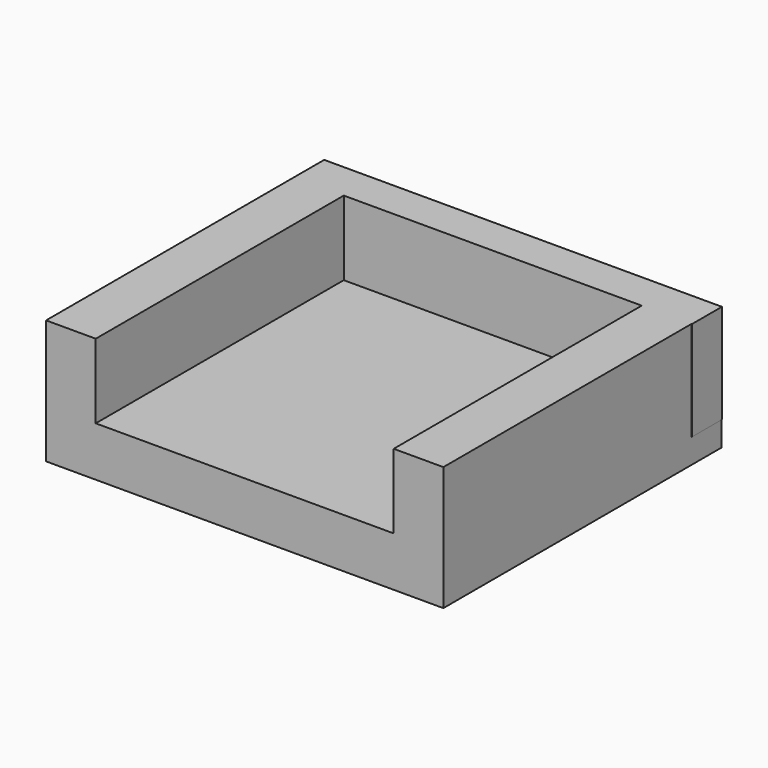
from build123d import *

# Parameters (mm, degrees)
F0_W     = 25.4
F0_H     = 25.4
F0_W_2   = 152.4
F0_H_2   = 38.1
F1_DEPTH = 177.8
F2_W     = 203.2
F2_H     = 19.2293866986
F3_DEPTH = 50.8


# Not quite as in the source:
# - a feature names something its author has since deleted; it is built from what else it names


with BuildPart() as f1:
    # F0 (on Front) → F1 (new body)
    with BuildSketch(Plane.XZ):
        with Locations((-88.9, 0)):
            Rectangle(F0_W, F0_H)
        Rectangle(F0_W_2, F0_H)
        with Locations((88.9, 0)):
            Rectangle(F0_W, F0_H)
        with Locations((88.9, 31.75)):
            Rectangle(F0_W, F0_H_2)
        with Locations((-88.9, 31.75)):
            Rectangle(F0_W, F0_H_2)
    extrude(amount=F1_DEPTH)

    # F2 (on Top) → F3 (join)
    with BuildSketch(Plane.XY):
        with Locations((0.2353874207, -9.6146933493)):
            Rectangle(F2_W, F2_H)
    extrude(amount=F3_DEPTH)


solid = f1.part
